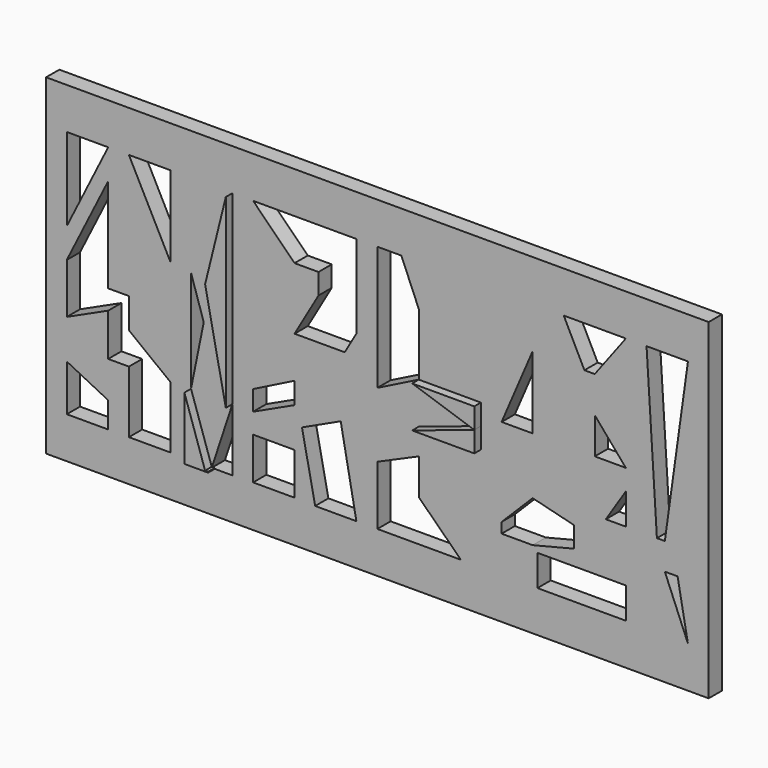
from build123d import *

# Parameters (mm, degrees)
F1_W     = 203.2
F1_H     = 101.6
F2_DEPTH = 5.08
F4_W     = 12.7
F4_H     = 12.9032718343
F4_W_2   = 27.1084083955
F4_H_2   = 9.525
F6_DEPTH = 6.35
F7_DEPTH = 6.35
F8_DEPTH = 2.54


with BuildPart() as f2:
    # F1 (on Front) → F2 (new body)
    with BuildSketch(Plane.XZ):
        with Locations((101.6, 50.8)):
            Rectangle(F1_W, F1_H)
    extrude(amount=-F2_DEPTH)

    # F4 (on face) → F6 (cut)
    with BuildSketch(Plane.XZ):
        Polygon((6.35, 88.9), (6.35, 63.4896950778), (19.05, 88.9), align=None)
        Polygon((38.1, 88.9), (25.4, 88.9), (38.1, 64.2026114812), align=None)
        Polygon((19.05, 79.7638625923), (6.35, 54.3535576701), (6.35, 38.9748217106), (19.05, 44.7899766155), (19.05, 31.75), (25.4, 31.75), (25.4, 12.7), (38.1, 12.7), (38.1, 31.75), (25.3980111729, 41.5485496718), (25.4, 50.8), (19.05, 50.8), align=None)
        Polygon((19.05, 20.5959144004), (6.35, 26.9433392146), (6.35, 12.7), (19.05, 12.7), align=None)
        Polygon((48.3517487947, 51.1962487751), (44.45, 63.2637151304), (44.45, 31.964471331), align=None)
        Polygon((57.15, 12.7), (57.15, 31.964471331), (50.8, 12.7), align=None)
        with Locations((69.85, 19.3217204115)):
            Rectangle(F4_W, F4_H)
        Polygon((90.3535660462, 38.1168511729), (78.4824932634, 32.6018280187), (82.5201821204, 12.7), (95.1624735994, 12.7), align=None)
        Polygon((76.2, 44.45), (63.5, 38.0811007293), (63.5, 31.964471331), (76.2, 37.8645947099), align=None)
        Polygon((95.25, 88.9), (63.5, 88.9), (76.2, 76.2), (83.5397814848, 76.2), (83.5397814848, 69.85), (76.2, 57.15), (91.5801092576, 57.15), (95.25, 63.5), align=None)
        Polygon((101.6, 50.8), (114.3, 57.15), (114.3, 76.2), (108.9507660084, 88.9), (101.6, 88.9), align=None)
        Polygon((114.3, 36.4221383274), (101.6, 30.8501303583), (101.6, 12.7), (127.2270479083, 12.7), (114.3, 25.4), align=None)
        Polygon((149.225, 53.975), (149.225, 76.2), (139.7, 53.975), align=None)
        Polygon((177.8, 88.9), (158.75, 88.9), (165.1, 76.2), (168.275, 76.2), align=None)
        Polygon((149.225, 36.5125), (139.7, 26.9875), (139.7, 23.8125), (149.225, 23.8125), (161.925, 26.9875), (161.925, 33.3375), align=None)
        with Locations((164.2457958023, 17.4625)):
            Rectangle(F4_W_2, F4_H_2)
    extrude(amount=-F6_DEPTH, mode=Mode.SUBTRACT)

    # F4 (on face) + F5 (on face) → F7 (cut)
    with BuildSketch(Plane.XZ):
        Polygon((187.325, 88.9), (187.325, 38.1), (189.7574476064, 38.1), (196.85, 88.9), align=None)
        Polygon((193.675, 29.845), (189.7574476064, 29.845), (196.85, 12.7), align=None)
        Polygon((177.8, 38.1), (177.8, 47.625), (171.658446914, 38.1), align=None)
    with BuildSketch(Plane.XZ):
        Polygon((177.8, 53.975), (168.275, 65.0875), (168.275, 53.975), align=None)
        Polygon((196.85, 88.9), (184.15, 88.9), (187.325, 38.1), (189.7574476064, 38.1), align=None)
    extrude(amount=-F7_DEPTH, mode=Mode.SUBTRACT)

    # F5 (on face) → F8 (join)
    with BuildSketch(Plane.XZ):
        Polygon((57.15, 88.9), (50.8, 63.2637151304), (57.15, 31.964471331), align=None)
    extrude(amount=F8_DEPTH)


with BuildPart() as f8:
    # F5 (on face) → F8, piece 2 (new body)
    with BuildSketch(Plane.XZ):
        Polygon((44.45, 31.964471331), (44.45, 12.7), (50.8, 12.7), (51.7085269504, 12.7), (51.7085269504, 12.954), (50.8, 12.954), align=None)
    extrude(amount=F8_DEPTH)


with BuildPart() as f8b:
    # F5 (on face) → F8, piece 3 (new body)
    with BuildSketch(Plane.XZ):
        Polygon((133.35, 57.15), (114.3, 57.15), (133.35, 50.8), align=None)
    extrude(amount=F8_DEPTH)


with BuildPart() as f8c:
    # F5 (on face) → F8, piece 4 (new body)
    with BuildSketch(Plane.XZ):
        Polygon((133.35, 44.45), (133.35, 50.8), (114.3, 44.45), align=None)
    extrude(amount=F8_DEPTH)


solid = Compound([f2.part, f8.part, f8b.part, f8c.part])
